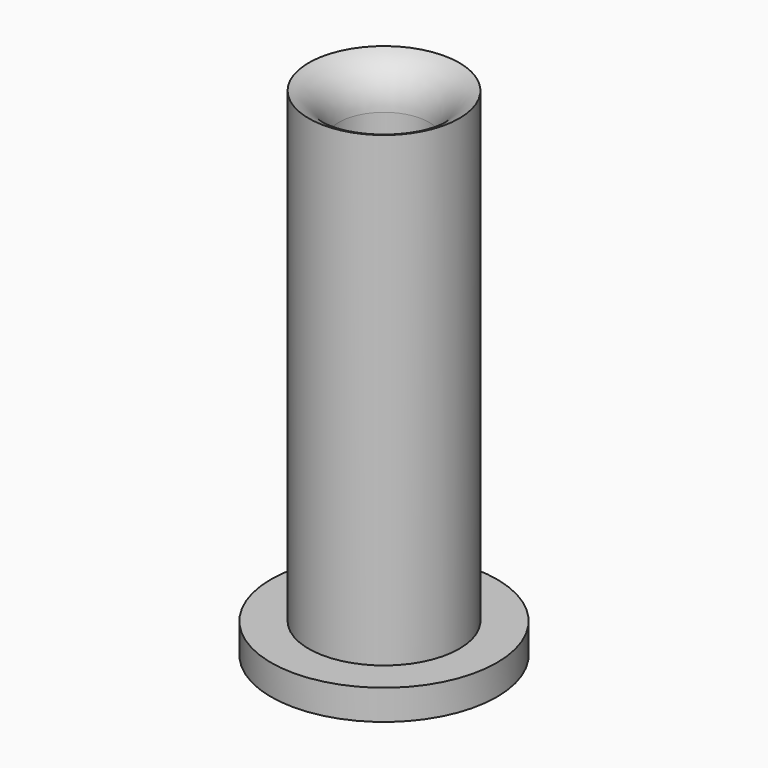
from build123d import *

# Parameters (mm, degrees)
F0_R     = 7.5
F0_R_2   = 5
F1_DEPTH = 2
F0_R_3   = 3
F2_DEPTH = 33


# Not quite as in the source:
# - a fillet or chamfer that OpenCascade refuses, or shapes differently, is made with other operations: its cross-section is extruded or revolved along the edge and cut away or added


with BuildPart() as f1:
    # F0 (on Top) → F1 (new body)
    with BuildSketch(Plane.XY):
        Circle(F0_R)
        Circle(F0_R_2, mode=Mode.SUBTRACT)
    extrude(amount=F1_DEPTH)

    # F0 (on Top) → F2 (join)
    with BuildSketch(Plane.XY):
        Circle(F0_R_2)
        Circle(F0_R_3, mode=Mode.SUBTRACT)
    extrude(amount=F2_DEPTH)

    # F3: fillet of radius 3 on 2 edges, made by hand

    # F3_s1 → F3_t2 (revolve, cut)
    with BuildSketch(Plane.XZ):
        with BuildLine():
            ThreePointArc((6, 0), (3.8786796564, 0.8786796564), (3, 3))
            Line((3, 3), (3, 0))
            Line((3, 0), (6, 0))
        make_face()
    revolve(axis=Axis((0, 0, 0), (0, 0, 1)), mode=Mode.SUBTRACT)

    # F3_s3 → F3_t4 (revolve, cut)
    with BuildSketch(Plane.XZ):
        with BuildLine():
            ThreePointArc((3, 30.1715728753), (3.5505102572, 31.9036236828), (5, 33))
            Line((5, 33), (3, 33))
            Line((3, 33), (3, 30.1715728753))
        make_face()
    revolve(axis=Axis((0, 0, 33), (0, 0, 1)), mode=Mode.SUBTRACT)


solid = f1.part
